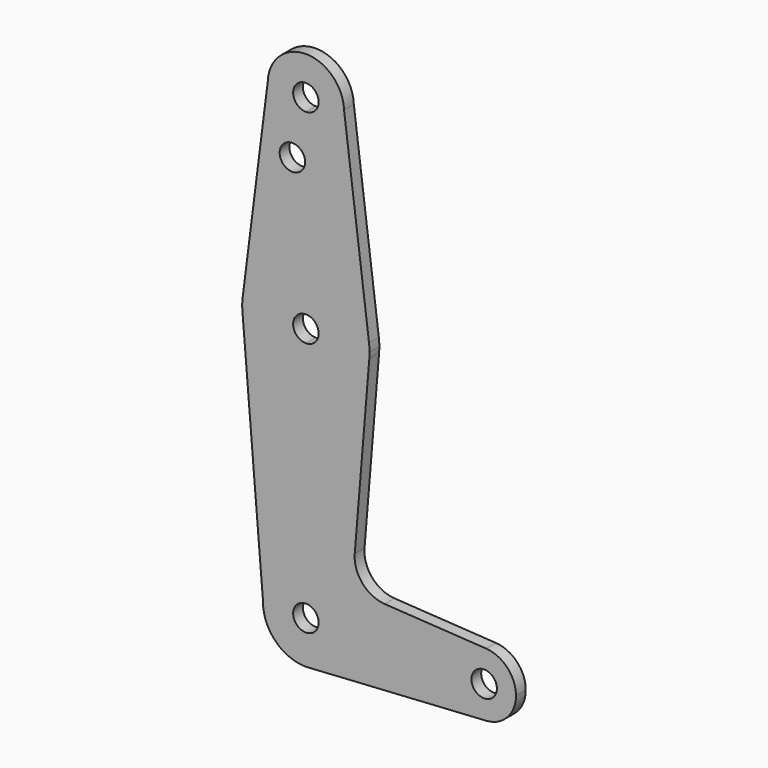
from build123d import *

# Parameters (mm, degrees)
F0_R     = 3.175
F1_DEPTH = 3.048


# Not quite as in the source:
# - ends of sketch curves that miss each other by under 0.0002 mm in the source are joined


with BuildPart() as f1:
    # F0 (on Front) → F1 (new body)
    with BuildSketch(Plane.XZ):
        with BuildLine():
            ThreePointArc((0, -42.9560914541), (7.5600620245, -46.0875716771), (10.6915422474, -53.6476337016))
            Line((10.6915422474, -53.6476337016), (36.5125, -53.6476337016))
            ThreePointArc((36.5125, -53.6476337016), (39.0126759444, -47.8649515069), (44.9381789581, -45.725160126))
            Line((44.9381789581, -45.725160126), (19.6163710563, -44.1648504083))
            ThreePointArc((19.6163710563, -44.1648504083), (14.0942781367, -41.4328681595), (12.1820328049, -35.5762005907))
            Line((12.1820328049, -35.5762005907), (15.8212777121, 8.5474538872))
            ThreePointArc((15.8212777121, 8.5474538872), (10.7540722598, -1.825200003), (0, -6.0226337016))
            Line((0, -6.0226337016), (0, -42.9560914541))
        make_face()
        with BuildLine():
            ThreePointArc((-10.690047341, -53.4688503814), (-7.4965860966, -46.0246242876), (0, -42.9560914541))
            Line((0, -42.9560914541), (0, -6.0226337016))
            ThreePointArc((0, -6.0226337016), (-10.7540722823, -1.8251999914), (-15.8212777256, 8.5474539313))
            Line((-15.8212777256, 8.5474539313), (-10.690047341, -53.4688503814))
        make_face()
        with BuildLine():
            Line((10.6915422474, -53.6476337016), (3.175, -53.6476337016))
            ThreePointArc((3.175, -53.6476337016), (-2.2450640303, -55.8926977318), (0, -50.4726337016))
            Line((0, -50.4726337016), (0, -42.9560914541))
            ThreePointArc((0, -42.9560914541), (-7.4965860966, -46.0246242876), (-10.690047341, -53.4688503814))
            ThreePointArc((-10.690047341, -53.4688503814), (-7.6230094139, -61.1442197982), (0, -64.339175949))
            Line((0, -64.339175949), (1.3126312246, -64.2582922531))
            ThreePointArc((1.3126312246, -64.2582922531), (8.0107155679, -60.7284183839), (10.6915422474, -53.6476337016))
        make_face()
        with BuildLine():
            ThreePointArc((0, -50.4726337016), (2.2450640303, -51.4025696713), (3.175, -53.6476337016))
            Line((3.175, -53.6476337016), (10.6915422474, -53.6476337016))
            ThreePointArc((10.6915422474, -53.6476337016), (7.5600620245, -46.0875716771), (0, -42.9560914541))
            Line((0, -42.9560914541), (0, -50.4726337016))
        make_face()
        with BuildLine():
            Line((36.5125, -53.6476337016), (10.6915422474, -53.6476337016))
            ThreePointArc((10.6915422474, -53.6476337016), (8.0107155679, -60.7284183839), (1.3126312246, -64.2582922531))
            Line((1.3126312246, -64.2582922531), (44.9381789581, -61.5701072771))
            ThreePointArc((44.9381789581, -61.5701072771), (39.0126759444, -59.4303158963), (36.5125, -53.6476337016))
        make_face()
        with BuildLine():
            ThreePointArc((44.9381789581, -45.725160126), (39.0126759444, -47.8649515069), (36.5125, -53.6476337016))
            ThreePointArc((36.5125, -53.6476337016), (39.0126759444, -59.4303158963), (44.9381789581, -61.5701072771))
            ThreePointArc((44.9381789581, -61.5701072771), (50.2326821947, -59.0849577571), (52.3875, -53.6476337016))
            ThreePointArc((52.3875, -53.6476337016), (50.2326821947, -48.210309646), (44.9381789581, -45.725160126))
        make_face()
        with BuildLine():
            ThreePointArc((47.625, -53.6476337016), (44.45, -56.8226337016), (41.275, -53.6476337016))
            ThreePointArc((41.275, -53.6476337016), (44.45, -50.4726337016), (47.625, -53.6476337016))
        make_face(mode=Mode.SUBTRACT)
        with BuildLine():
            ThreePointArc((-15.8212777256, 8.5474539313), (-10.7540722823, -1.8251999914), (0, -6.0226337016))
            Line((0, -6.0226337016), (0, 6.6773662984))
            ThreePointArc((0, 6.6773662984), (-3.1750000049, 9.8523662984), (0, 13.0273662984))
            Line((0, 13.0273662984), (0, 25.7273662984))
            ThreePointArc((0, 25.7273662984), (-10.2345652868, 21.9878225524), (-15.6473851089, 12.5309787019))
            Line((-15.6473851089, 12.5309787019), (-15.8212782601, 11.157272185))
            ThreePointArc((-15.8212782601, 11.157272185), (-15.8750000049, 9.8523630471), (-15.8212777256, 8.5474539313))
        make_face()
        with BuildLine():
            Line((0, 6.6773662984), (0, -6.0226337016))
            ThreePointArc((0, -6.0226337016), (10.7540722598, -1.825200003), (15.8212777121, 8.5474538872))
            ThreePointArc((15.8212777121, 8.5474538872), (15.8615637383, 9.1993574002), (15.8749999951, 9.8523662984))
            ThreePointArc((15.8749999951, 9.8523662984), (15.843418635, 10.8532213331), (15.7488002092, 11.8500942118))
            ThreePointArc((15.7488002092, 11.8500942118), (10.4952773724, 21.7630664363), (0, 25.7273662984))
            Line((0, 25.7273662984), (0, 13.0273662984))
            ThreePointArc((0, 13.0273662984), (2.2450640271, 12.097430327), (3.1749999951, 9.8523662984))
            ThreePointArc((3.1749999951, 9.8523662984), (2.2450640271, 7.6073022699), (0, 6.6773662984))
        make_face()
        with BuildLine():
            ThreePointArc((0, 25.7273662984), (10.4952773724, 21.7630664363), (15.7488002092, 11.8500942118))
            Line((15.7488002092, 11.8500942118), (9.5202989573, 60.9515865588))
            ThreePointArc((9.5202989573, 60.9515865588), (9.5238246668, 60.801994892), (9.525, 60.6523662984))
            ThreePointArc((9.525, 60.6523662984), (6.7351920908, 53.9171742076), (0, 51.1273662984))
            Line((0, 51.1273662984), (0, 25.7273662984))
        make_face()
        with BuildLine():
            Line((-9.5210262398, 60.9274741696), (-15.6473851089, 12.5309787019))
            ThreePointArc((-15.6473851089, 12.5309787019), (-10.2345652868, 21.9878225524), (0, 25.7273662984))
            Line((0, 25.7273662984), (0, 51.1273662984))
            ThreePointArc((0, 51.1273662984), (-6.8317650528, 54.0151521793), (-9.5210262398, 60.9274741696))
        make_face()
        with Locations((-3.3664405459, 46.3775662984)):
            Circle(F0_R, mode=Mode.SUBTRACT)
        with BuildLine():
            ThreePointArc((9.5202989573, 60.9515865588), (-0.0120616774, 70.1773586615), (-9.5210262398, 60.9274741696))
            ThreePointArc((-9.5210262398, 60.9274741696), (-6.8317650528, 54.0151521793), (0, 51.1273662984))
            ThreePointArc((0, 51.1273662984), (6.7351920908, 53.9171742076), (9.525, 60.6523662984))
            ThreePointArc((9.525, 60.6523662984), (9.5238246668, 60.801994892), (9.5202989573, 60.9515865588))
        make_face()
        with BuildLine():
            ThreePointArc((3.175, 60.6523662984), (2.2450640303, 58.4073022682), (0, 57.4773662984))
            ThreePointArc((0, 57.4773662984), (-2.2450640303, 62.8974303287), (3.175, 60.6523662984))
        make_face(mode=Mode.SUBTRACT)
    extrude(amount=F1_DEPTH)


solid = f1.part
